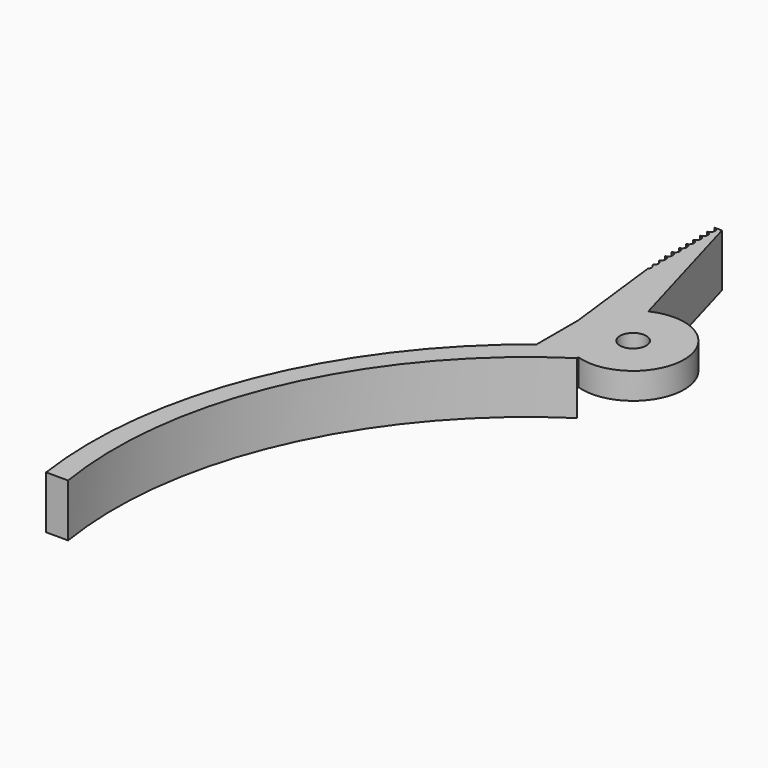
from build123d import *

# Parameters (mm, degrees)
F0_R     = 1.905
F1_DEPTH = 3.81
F2_DEPTH = 3.81
F4_DEPTH = 7.621


# Not quite as in the source:
# - a feature names something its author has since deleted; it is built from what else it names


with BuildPart() as f1:
    # F0 (on Top) → F1 (new body)
    with BuildSketch(Plane.XY):
        with BuildLine():
            ThreePointArc((-28.4269883335, -66.4172298291), (-24.0943230698, -32.9852682882), (-2.3028327904, -7.2637016141))
            Line((-2.3028327904, -7.2637016141), (-7.943934761, -7.4889131964))
            ThreePointArc((-7.943934761, -7.4889131964), (-27.6668151141, -33.7839124183), (-31.6019883335, -66.4172298291))
            Line((-31.6019883335, -66.4172298291), (-28.4269883335, -66.4172298291))
        make_face()
        with BuildLine():
            ThreePointArc((-2.3028327904, -7.2637016141), (-7.6043838567, -0.4875922071), (-3.211656147, 6.9101132258))
            Line((-3.211656147, 6.9101132258), (-10.16, 31.3176262796))
            Line((-10.16, 31.3176262796), (-10.16, 18.6176262796))
            Line((-10.16, 18.6176262796), (-7.943934761, 0))
            Line((-7.943934761, 0), (-7.943934761, -7.4889131964))
            Line((-7.943934761, -7.4889131964), (-2.3028327904, -7.2637016141))
        make_face()
        with BuildLine():
            ThreePointArc((7.366, 0), (3.9446061685, 6.2207747247), (-3.1412055867, 6.6626408775))
            ThreePointArc((-3.1412055867, 6.6626408775), (-7.3521647617, -0.4512530518), (-2.3028327904, -6.9967790546))
            ThreePointArc((-2.3028327904, -6.9967790546), (4.3182918883, -5.9674375713), (7.366, 0))
        make_face()
        Circle(F0_R, mode=Mode.SUBTRACT)
        with BuildLine():
            Line((-3.1412055867, 6.6626408775), (-3.211656147, 6.9101132258))
            ThreePointArc((-3.211656147, 6.9101132258), (-7.6043838567, -0.4875922071), (-2.3028327904, -7.2637016141))
            Line((-2.3028327904, -7.2637016141), (-2.3028327904, -6.9967790546))
            ThreePointArc((-2.3028327904, -6.9967790546), (-7.3521647617, -0.4512530518), (-3.1412055867, 6.6626408775))
        make_face()
    extrude(amount=F1_DEPTH)

    # F0 (on Top) → F2 (join)
    with BuildSketch(Plane.XY):
        with BuildLine():
            ThreePointArc((-2.3028327904, -7.2637016141), (-7.6043838567, -0.4875922071), (-3.211656147, 6.9101132258))
            Line((-3.211656147, 6.9101132258), (-10.16, 31.3176262796))
            Line((-10.16, 31.3176262796), (-10.16, 18.6176262796))
            Line((-10.16, 18.6176262796), (-7.943934761, 0))
            Line((-7.943934761, 0), (-7.943934761, -7.4889131964))
            Line((-7.943934761, -7.4889131964), (-2.3028327904, -7.2637016141))
        make_face()
        with BuildLine():
            ThreePointArc((-28.4269883335, -66.4172298291), (-24.0943230698, -32.9852682882), (-2.3028327904, -7.2637016141))
            Line((-2.3028327904, -7.2637016141), (-7.943934761, -7.4889131964))
            ThreePointArc((-7.943934761, -7.4889131964), (-27.6668151141, -33.7839124183), (-31.6019883335, -66.4172298291))
            Line((-31.6019883335, -66.4172298291), (-28.4269883335, -66.4172298291))
        make_face()
    extrude(amount=-F2_DEPTH)

    # F3 (on face) → F4 (cut, through all)
    with BuildSketch(Plane.XY.offset(3.81)):
        with BuildLine():
            Line((-10.16, 27.284329945), (-10.1133690513, 27.284329945))
            ThreePointArc((-10.1133690513, 27.284329945), (-10.1366687719, 27.2856156574), (-10.16, 27.2860444212))
            Line((-10.16, 27.2860444212), (-10.16, 27.284329945))
        make_face()
        with BuildLine():
            Line((-10.16, 28.5560444212), (-10.16, 27.2860444212))
            ThreePointArc((-10.16, 27.2860444212), (-9.7109871939, 27.4720316151), (-9.525, 27.9210444212))
            ThreePointArc((-9.525, 27.9210444212), (-9.7109871939, 28.3700572272), (-10.16, 28.5560444212))
        make_face()
        with BuildLine():
            Line((-10.1133690513, 27.284329945), (-9.0117990451, 27.284329945))
            Line((-9.0117990451, 27.284329945), (-10.16, 31.3176262796))
            Line((-10.16, 31.3176262796), (-10.16, 28.5560444212))
            ThreePointArc((-10.16, 28.5560444212), (-9.7109871939, 28.3700572272), (-9.525, 27.9210444212))
            ThreePointArc((-9.525, 27.9210444212), (-9.7109871939, 27.4720316151), (-10.16, 27.2860444212))
            ThreePointArc((-10.16, 27.2860444212), (-10.1366687719, 27.2856156574), (-10.1133690513, 27.284329945))
        make_face()
        with BuildLine():
            ThreePointArc((-9.525, 19.0310444212), (-9.7109871939, 19.4800572272), (-10.16, 19.6660444212))
            Line((-10.16, 19.6660444212), (-10.16, 18.6176262796))
            Line((-10.16, 18.6176262796), (-10.1336899082, 18.3965897112))
            ThreePointArc((-10.1336899082, 18.3965897112), (-9.7017795791, 18.5914320398), (-9.525, 19.0310444212))
        make_face()
        with BuildLine():
            Line((-10.16, 27.284329945), (-10.16, 26.0160444212))
            ThreePointArc((-10.16, 26.0160444212), (-9.7109871939, 26.2020316151), (-9.525, 26.6510444212))
            ThreePointArc((-9.525, 26.6510444212), (-9.6947927062, 27.0832563759), (-10.1133690513, 27.284329945))
            Line((-10.1133690513, 27.284329945), (-10.16, 27.284329945))
        make_face()
        with BuildLine():
            Line((-10.16, 26.0160444212), (-10.16, 24.7460444212))
            ThreePointArc((-10.16, 24.7460444212), (-9.7109871939, 24.9320316151), (-9.525, 25.3810444212))
            ThreePointArc((-9.525, 25.3810444212), (-9.7109871939, 25.8300572272), (-10.16, 26.0160444212))
        make_face()
        with BuildLine():
            Line((-10.16, 24.7460444212), (-10.16, 23.4760444212))
            ThreePointArc((-10.1600000026, 23.4760444212), (-9.7109871948, 23.6620316142), (-9.525, 24.1110444212))
            ThreePointArc((-9.525, 24.1110444212), (-9.7109871939, 24.5600572272), (-10.16, 24.7460444212))
        make_face()
        with BuildLine():
            Line((-10.16, 23.4760444212), (-10.16, 22.2060444212))
            ThreePointArc((-10.16, 22.2060444212), (-9.7109871939, 22.3920316151), (-9.525, 22.8410444212))
            ThreePointArc((-9.525, 22.8410444212), (-9.7109871948, 23.2900572282), (-10.1600000026, 23.4760444212))
        make_face()
        with BuildLine():
            Line((-10.16, 22.2060444212), (-10.16, 20.9360444212))
            ThreePointArc((-10.16, 20.9360444212), (-9.7109871939, 21.1220316151), (-9.525, 21.5710444212))
            ThreePointArc((-9.525, 21.5710444212), (-9.7109871939, 22.0200572272), (-10.16, 22.2060444212))
        make_face()
        with BuildLine():
            Line((-10.16, 20.9360444212), (-10.16, 19.6660444212))
            ThreePointArc((-10.16, 19.6660444212), (-9.7109871939, 19.8520316151), (-9.525, 20.3010444212))
            ThreePointArc((-9.525, 20.3010444212), (-9.7109871939, 20.7500572272), (-10.16, 20.9360444212))
        make_face()
        with BuildLine():
            Line((-10.1335594504, 18.3954937079), (-9.9853706378, 17.1505285853))
            ThreePointArc((-9.9853706378, 17.1505285853), (-9.6529917925, 17.3787256046), (-9.525, 17.7610444212))
            ThreePointArc((-9.525, 17.7610444212), (-9.7017343843, 18.20060969), (-10.1335594504, 18.3954937079))
        make_face()
        with BuildLine():
            Line((-9.9793324764, 17.099800732), (-9.8414839109, 15.941706182))
            ThreePointArc((-9.8414839109, 15.941706182), (-9.6097806271, 16.1740528729), (-9.525, 16.4910444212))
            ThreePointArc((-9.525, 16.4910444212), (-9.6511046878, 16.8708477404), (-9.9793324764, 17.099800732))
        make_face()
        with BuildLine():
            ThreePointArc((-9.7032002185, 14.7799560404), (-9.5712331271, 14.9831819202), (-9.525, 15.2210444212))
            ThreePointArc((-9.525, 15.2210444212), (-9.6034746489, 15.5268295313), (-9.8195024679, 15.7570354945))
            Line((-9.8195024679, 15.7570354945), (-9.7032002185, 14.7799560404))
        make_face()
    extrude(amount=-F4_DEPTH, mode=Mode.SUBTRACT)


solid = f1.part
